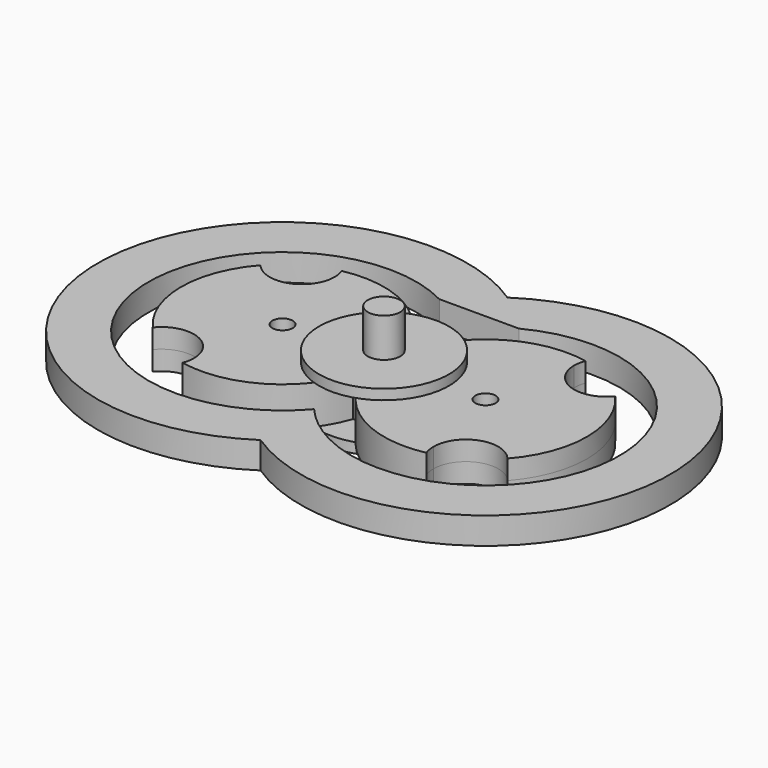
from build123d import *

# Parameters (mm, degrees)
F0_R          = 5
F1_DEPTH      = 9.6
F2_DEPTH      = 12.5
F3_W          = 8
F3_H          = 19.2
F3_W_2        = 16
F7_DEPTH      = 6.6
F7_DEPTH_BACK = 6.6


# Not quite as in the source:
# - a feature names something its author has since deleted; it is built from what else it names


with BuildPart() as f1:
    # F0 (on Top) → F1 (new body, symmetric)
    with BuildSketch(Plane.XY):
        with BuildLine():
            ThreePointArc((-2.56, -15.7938722294), (-16, 0), (-2.56, 15.7938722294))
            ThreePointArc((-2.56, 15.7938722294), (-25, 43.3012701892), (-60.0421054252, 48.9811812703))
            ThreePointArc((-60.0421054252, 48.9811812703), (-59.2626826747, 46.1886294328), (-59, 43.3012701892))
            ThreePointArc((-59, 43.3012701892), (-69.6318677921, 28.2286739763), (-87.3978945748, 33.1873090408))
            ThreePointArc((-87.3978945748, 33.1873090408), (-100, 0), (-87.3978945748, -33.1873090408))
            ThreePointArc((-87.3978945748, -33.1873090408), (-69.6318677921, -28.2286739763), (-59, -43.3012701892))
            ThreePointArc((-59, -43.3012701892), (-59.2626826747, -46.1886294328), (-60.0421054252, -48.9811812703))
            ThreePointArc((-60.0421054252, -48.9811812703), (-25, -43.3012701892), (-2.56, -15.7938722294))
        make_face()
        with Locations((-50, 0)):
            Circle(F0_R, mode=Mode.SUBTRACT)
    extrude(amount=F1_DEPTH, both=True)


with BuildPart() as f2:
    # F0 (on Top) → F2 (new body, symmetric)
    with BuildSketch(Plane.XY):
        with BuildLine():
            ThreePointArc((-2.56, -15.7938722294), (-0.644149283, -8), (0, 0))
            ThreePointArc((0, 0), (-0.644149283, 8), (-2.56, 15.7938722294))
            ThreePointArc((-2.56, 15.7938722294), (-16, 0), (-2.56, -15.7938722294))
        make_face()
    extrude(amount=F2_DEPTH, both=True)


with BuildPart() as f4:
    # F3 (on Front) → F4 (revolve)
    with BuildSketch(Plane.XZ):
        Polygon((0, 9.6), (0, 12.5), (0, 14.6), (-8, 14.6), (-32, 14.6), (-32, 9.6), (-16, 9.6), align=None)
        with Locations((-4, 24.2)):
            Rectangle(F3_W, F3_H)
        with Locations((-8, 0)):
            Rectangle(F3_W_2, F3_H)
        Polygon((0, -12.5), (0, -9.6), (-16, -9.6), (-32, -9.6), (-32, -14.6), (0, -14.6), align=None)
    revolve(axis=Axis((0, 0, 0), (0, 0, -1)))


with BuildPart() as f5_1:
    # F5: instance of F1
    add(f1.part.mirror(Plane.YZ))


with BuildPart() as f7:
    # F6 (on Top) → F7 (new body, two sides)
    with BuildSketch(Plane.XY) as f7_sk:
        with BuildLine():
            ThreePointArc((0, 76.0328876211), (-141, 0), (0, -76.0328876211))
            ThreePointArc((0, -76.0328876211), (141, 0), (0, 76.0328876211))
        make_face()
        with BuildLine():
            ThreePointArc((-19.625, -58.5948749892), (-116, 0), (-19.625, 58.5948749892))
            Line((-19.625, 58.5948749892), (19.625, 58.5948749892))
            ThreePointArc((19.625, 58.5948749892), (115.9996126841, 0.2261095817), (20.0271913422, -58.8016219263))
            ThreePointArc((20.0271913422, -58.8016219263), (19.8259185969, -58.6985929259), (19.625, -58.5948749892))
            ThreePointArc((19.625, -58.5948749892), (9.070759043, -51.7764158153), (0, -43.0813184571))
            ThreePointArc((0, -43.0813184571), (-9.070759043, -51.7764158153), (-19.625, -58.5948749892))
        make_face(mode=Mode.SUBTRACT)
    extrude(amount=F7_DEPTH)
    extrude(f7_sk.sketch, amount=-F7_DEPTH_BACK)


solid = Compound([f1.part, f2.part, f4.part, f5_1.part, f7.part])
